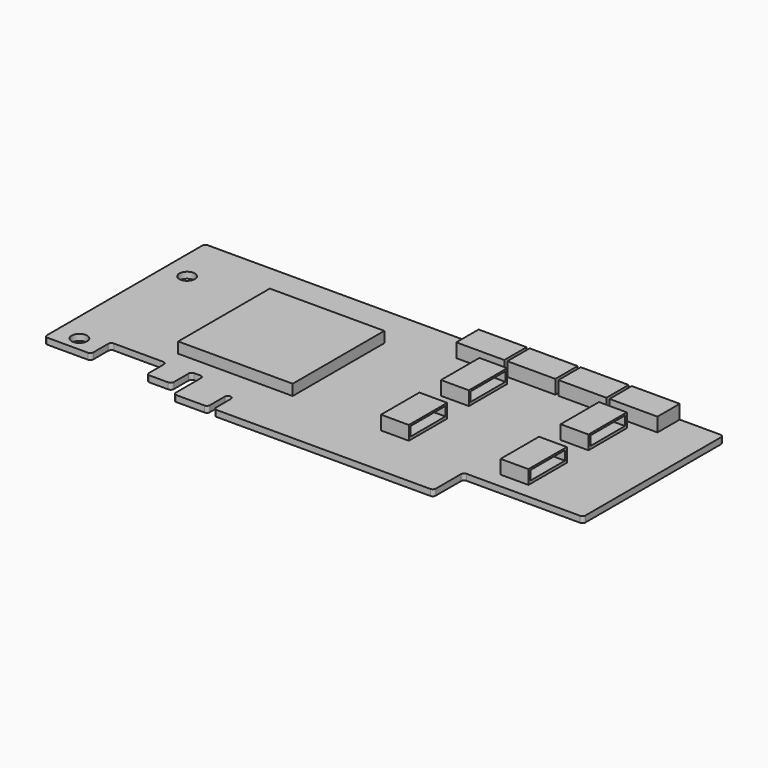
from build123d import *

# Parameters (mm, degrees)
F0_R          = 2.5
F1_DEPTH      = 2
F3_R          = 0.99999
F2_W          = 15.5
F2_H          = 9
F2_W_2        = 9
F2_H_2        = 15.5
F2_W_3        = 37
F2_H_3        = 37
F4_DEPTH      = 0.5
F5_DEPTH      = 0.5
F6_DEPTH      = 5
F7_W          = 14
F7_H          = 3
F8_DEPTH      = 107.3565227488
F8_DEPTH_BACK = 60.2954772512
F9_W          = 13
F9_H          = 3
F10_DEPTH     = 5
F11_DEPTH     = 4


# Not quite as in the source:
# - a fillet or chamfer is up to 0.001 mm smaller than in the source, because OpenCascade refuses the exact size


with BuildPart() as f1:
    # F0 (on Top) → F1 (new body)
    with BuildSketch(Plane.XY):
        Polygon((83.825, -24.3705166107), (83.825, 32.3705166107), (-83.825, 32.3705166107), (-83.825, -32.3705166107), (-68.825, -32.3705166107), (-68.825, -24.3705166107), (-50.825, -24.3705166107), (-50.825, -32.3705166107), (-42.825, -32.3705166107), (-42.825, -24.3705166107), (-38.825, -24.3705166107), (-38.825, -36.5294833893), (-27.825, -36.5294833893), (-27.825, -28.5294833893), (-25.825, -28.5294833893), (-25.825, -36.5294833893), (45.175, -36.5294833893), (45.175, -24.3705166107), align=None)
        with Locations((-76.325, -27.6294833893)):
            Circle(F0_R, mode=Mode.SUBTRACT)
        with Locations((-76.325, 15.8705166107)):
            Circle(F0_R, mode=Mode.SUBTRACT)
    extrude(amount=F1_DEPTH)

    # F3 (radius 1 in the source; OpenCascade refuses exactly that, so slightly less here)
    f3_edges = [f1.edges().sort_by_distance(p)[0] for p in [
        (-83.825, -32.370517, 1),
        (-68.825, -32.370517, 1),
        (-68.825, -24.370517, 1),
        (-50.825, -32.370517, 1),
        (-42.825, -32.370517, 1),
        (-42.825, -24.370517, 1),
        (-38.825, -36.529483, 1),
        (-27.825, -36.529483, 1),
        (-27.825, -28.529483, 1),
        (-25.825, -36.529483, 1),
        (83.825, -24.370517, 1),
        (45.175, -24.370517, 1),
        (45.175, -36.529483, 1),
        (83.825, 32.370517, 1),
        (-83.825, 32.370517, 1),
        (-50.825, -24.370517, 1),
        (-38.825, -24.370517, 1),
        (-25.825, -28.529483, 1),
    ]]
    fillet(f3_edges, radius=F3_R)

    # F2 (on face) → F4 (cut)
    with BuildSketch(Plane.XY.offset(2)):
        with Locations((-70.075, 27.8705166107)):
            Rectangle(F2_W, F2_H)
        with Locations((-53.575, 27.8705166107)):
            Rectangle(F2_W, F2_H)
        with Locations((-37.075, 27.8705166107)):
            Rectangle(F2_W, F2_H)
        with Locations((-20.575, 27.8705166107)):
            Rectangle(F2_W, F2_H)
        with Locations((-4.075, 27.8705166107)):
            Rectangle(F2_W, F2_H)
        with Locations((12.425, 27.8705166107)):
            Rectangle(F2_W, F2_H)
        with Locations((28.925, 27.8705166107)):
            Rectangle(F2_W, F2_H)
        with Locations((45.425, 27.8705166107)):
            Rectangle(F2_W, F2_H)
        with Locations((61.925, 27.8705166107)):
            Rectangle(F2_W, F2_H)
        with Locations((57.675, 12.6205166107)):
            Rectangle(F2_W_2, F2_H_2)
        with Locations((57.675, -11.6205166107)):
            Rectangle(F2_W_2, F2_H_2)
        with Locations((19.0305227488, 12.6205166107)):
            Rectangle(F2_W_2, F2_H_2)
        with Locations((19.0305227488, -11.6205166107)):
            Rectangle(F2_W_2, F2_H_2)
        with Locations((-33.1395904124, -0.086670503)):
            Rectangle(F2_W_3, F2_H_3)
    extrude(amount=-F4_DEPTH, mode=Mode.SUBTRACT)

    # F5 (add, through all): faces of the model
    f5_faces = [f1.faces().sort_by_distance(p)[0] for p in [
        (-70.075, 27.8705166107, 1.5),
        (-53.575, 27.8705166107, 1.5),
        (-37.075, 27.8705166107, 1.5),
        (-20.575, 27.8705166107, 1.5),
        (-4.075, 27.8705166107, 1.5),
    ]]
    extrude(f5_faces, amount=F5_DEPTH)

    # F6 (add): faces of the model
    f6_faces = [f1.faces().sort_by_distance(p)[0] for p in [
        (12.425, 27.8705166107, 1.5),
        (28.925, 27.8705166107, 1.5),
        (45.425, 27.8705166107, 1.5),
        (61.925, 27.8705166107, 1.5),
        (19.0305227488, 12.6205166107, 1.5),
        (57.675, 12.6205166107, 1.5),
        (19.0305227488, -11.6205166107, 1.5),
        (57.675, -11.6205166107, 1.5),
    ]]
    extrude(f6_faces, amount=F6_DEPTH)

    # F7 (on face) → F8 (cut, two sides)
    with BuildSketch(Plane.YZ.offset(23.5305227488)) as f8_sk:
        with Locations((-11.6205166107, 4.4102044776)):
            Rectangle(F7_W, F7_H)
        with Locations((12.6205166107, 4.4102044776)):
            Rectangle(F7_W, F7_H)
    extrude(amount=-F8_DEPTH, mode=Mode.SUBTRACT)
    extrude(f8_sk.sketch, amount=F8_DEPTH_BACK, mode=Mode.SUBTRACT)

    # F9 (on face) → F10 (cut)
    with BuildSketch(Plane(origin=(0, 32.3705166107, 0), x_dir=(-1, 0, 0), z_dir=(0, 1, 0))):
        with Locations((-12.425, 4.25)):
            Rectangle(F9_W, F9_H)
        with Locations((-28.925, 4.25)):
            Rectangle(F9_W, F9_H)
        with Locations((-45.425, 4.25)):
            Rectangle(F9_W, F9_H)
        with Locations((-61.925, 4.25)):
            Rectangle(F9_W, F9_H)
    extrude(amount=-F10_DEPTH, mode=Mode.SUBTRACT)

    # F11 (add): a face of the model
    f11_faces = [f1.faces().sort_by_distance(p)[0] for p in [
        (-33.1395904124, -0.086670503, 1.5),
    ]]
    extrude(f11_faces, amount=F11_DEPTH)


solid = f1.part
